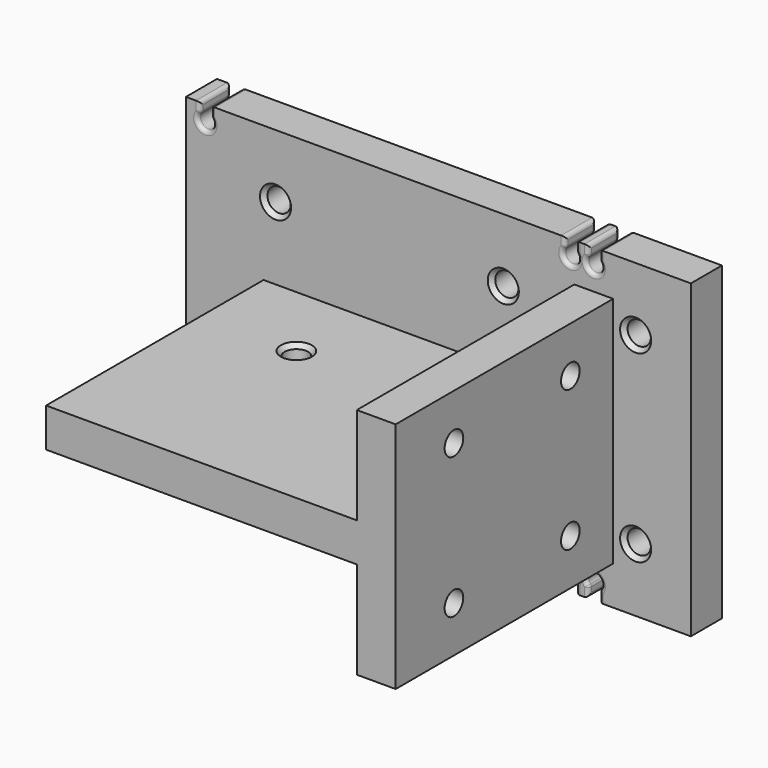
from build123d import *

# Parameters (mm, degrees)
F0_W                 = 10
F0_H                 = 20
F1_DEPTH             = 5
F2_R                 = 0.49999
F3_W                 = 40
F3_H                 = 2.5
F4_DEPTH             = 35
F8_D                 = 3
F8_CSINK_D           = 4
F8_CSINK_ANGLE       = 82
F8_ON_F7_D           = 3
F8_ON_F7_CSINK_D     = 4
F8_ON_F7_CSINK_ANGLE = 82
F8_ON_F6_D           = 3
F8_ON_F6_CSINK_D     = 4
F8_ON_F6_CSINK_ANGLE = 82


# Not quite as in the source:
# - a fillet or chamfer is up to 0.001 mm smaller than in the source, because OpenCascade refuses the exact size


with BuildPart() as f1:
    # F0 (on Front) → F1 (new body)
    with BuildSketch(Plane.XZ):
        with BuildLine():
            Line((-55, 0), (0, 0))
            Line((0, 0), (0, 20))
            Line((0, 20), (-1.7928932188, 20))
            Line((-1.7928932188, 20), (-1.7928932188, 18.6897154199))
            ThreePointArc((-1.7928932188, 18.6897154199), (-1.5761204675, 18.3652920711), (-1.5, 17.9826086387))
            ThreePointArc((-1.5, 17.9826086387), (-2.8826834324, 17.0587291062), (-3.2071067812, 18.6897154199))
            Line((-3.2071067812, 18.6897154199), (-3.2071067812, 20))
            Line((-3.2071067812, 20), (-4.7928932188, 20))
            Line((-4.7928932188, 20), (-4.7928932188, 18.6897154199))
            ThreePointArc((-4.7928932188, 18.6897154199), (-4.5761204675, 18.3652920711), (-4.5, 17.9826086387))
            ThreePointArc((-4.5, 17.9826086387), (-5.8826834324, 17.0587291062), (-6.2071067812, 18.6897154199))
            Line((-6.2071067812, 18.6897154199), (-6.2071067812, 20))
            Line((-6.2071067812, 20), (-51.7928932188, 20))
            Line((-51.7928932188, 20), (-51.7928932188, 18.6897154199))
            ThreePointArc((-51.7928932188, 18.6897154199), (-51.5761204675, 18.3652920711), (-51.5, 17.9826086387))
            ThreePointArc((-51.5, 17.9826086387), (-52.8826834324, 17.0587291062), (-53.2071067812, 18.6897154199))
            Line((-53.2071067812, 18.6897154199), (-53.2071067812, 20))
            Line((-53.2071067812, 20), (-55, 20))
            Line((-55, 20), (-55, 0))
        make_face()
        with Locations((5, 10)):
            Rectangle(F0_W, F0_H)
    extrude(amount=F1_DEPTH)

    # F2 (radius 0.5 in the source; OpenCascade refuses exactly that, so slightly less here)
    f2_edges = [f1.edges().sort_by_distance(p)[0] for p in [
        (-51.792893, -2.5, 20),
        (-51.792893, -2.5, 18.689715),
        (-51.792893, 0, 19.344858),
        (-51.792893, -5, 19.344858),
        (-53.207107, -2.5, 18.689715),
        (-52.5, 0, 16.982609),
        (-52.5, -5, 16.982609),
        (-53.207107, -2.5, 20),
        (-53.207107, 0, 19.344858),
        (-53.207107, -5, 19.344858),
        (-1.792893, -2.5, 20),
        (-1.792893, -2.5, 18.689715),
        (-1.792893, 0, 19.344858),
        (-1.792893, -5, 19.344858),
        (-3.207107, -2.5, 18.689715),
        (-3.207107, -2.5, 20),
        (-3.207107, 0, 19.344858),
        (-3.207107, -5, 19.344858),
        (-2.5, -5, 16.982609),
        (-2.5, 0, 16.982609),
        (-5.5, -5, 16.982609),
        (-5.5, 0, 16.982609),
        (-4.792893, -5, 19.344858),
        (-4.792893, -2.5, 20),
        (-6.207107, -2.5, 20),
        (-6.207107, -5, 19.344858),
        (-6.207107, 0, 19.344858),
        (-6.207107, -2.5, 18.689715),
        (-4.792893, -2.5, 18.689715),
        (-4.792893, 0, 19.344858),
    ]]
    fillet(f2_edges, radius=F2_R)

    # F3 (on face) → F4 (join)
    with BuildSketch(Plane.XZ.offset(5)):
        Polygon((-5, 0), (0, 0), (0, 15), (-5, 15), (-5, 2.5), align=None)
        with Locations((-25, 1.25)):
            Rectangle(F3_W, F3_H)
    extrude(amount=F4_DEPTH)

    # F8 (through all)
    with Locations(Plane.XZ.offset(5)):
        with Locations((-43.4641800821, 11.8344752118), (-14.1421612352, 11.8344752118), (2.8930022381, 11.8344752118)):
            CounterSinkHole(F8_D / 2, F8_CSINK_D / 2, counter_sink_angle=F8_CSINK_ANGLE)

    # F8 on F7 (through all)
    with Locations(Plane.XY.offset(2.5)):
        with Locations((-32.7726192772, -15.0109613314), (-14.8187577724, -15.0109613314)):
            CounterSinkHole(F8_ON_F7_D / 2, F8_ON_F7_CSINK_D / 2, counter_sink_angle=F8_ON_F7_CSINK_ANGLE)

    # F8 on F6 (through all)
    with Locations(Plane(origin=(-5, 0, 0), x_dir=(0, -1, 0), z_dir=(-1, 0, 0))):
        with Locations((11.8876462802, 9.0605169535), (30.620533973, 9.0605169535)):
            CounterSinkHole(F8_ON_F6_D / 2, F8_ON_F6_CSINK_D / 2, counter_sink_angle=F8_ON_F6_CSINK_ANGLE)

    # F9: F1 across face


with BuildPart() as f1_1:
    add(f1.part)
    add(f1.part.mirror(Plane(origin=(-22.490287011, -19.1094425862, 0), x_dir=(1, 0, 0), z_dir=(0, 0, -1))))


solid = f1_1.part
